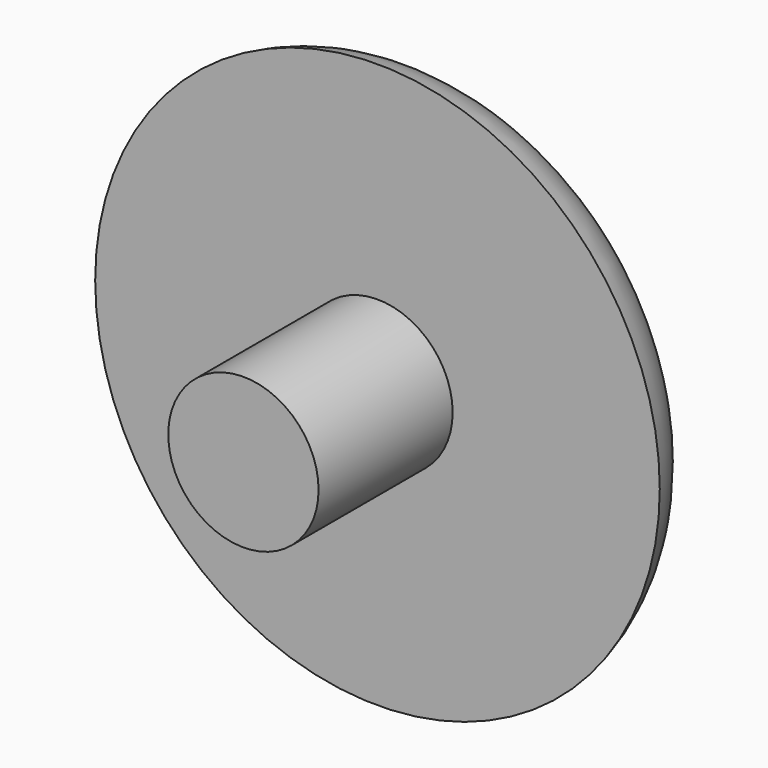
from build123d import *

# Parameters (mm, degrees)
F0_R     = 10.95
F1_DEPTH = 3
F2_R     = 2.915
F3_DEPTH = 6.5


# Not quite as in the source:
# - a fillet or chamfer that OpenCascade refuses, or shapes differently, is made with other operations: its cross-section is extruded or revolved along the edge and cut away or added


with BuildPart() as f1:
    # F0 (on Front) → F1 (new body)
    with BuildSketch(Plane.XZ):
        Circle(F0_R)
    extrude(amount=F1_DEPTH)

    # F2 (on face) → F3 (join)
    with BuildSketch(Plane.XZ.offset(3)):
        Circle(F2_R)
    extrude(amount=F3_DEPTH)

    # F4: fillet of radius 3.81 on 1 edges, made by hand

    # F4_s1 → F4_t2 (revolve, cut)
    with BuildSketch(Plane.XY):
        with BuildLine():
            ThreePointArc((10.95, -3), (9.6177045238, -0.843335206), (7.2270979062, 0))
            Line((7.2270979062, 0), (10.95, 0))
            Line((10.95, 0), (10.95, -3))
        make_face()
    revolve(axis=Axis((0, 0, 0), (0, -1, 0)), mode=Mode.SUBTRACT)


solid = f1.part
